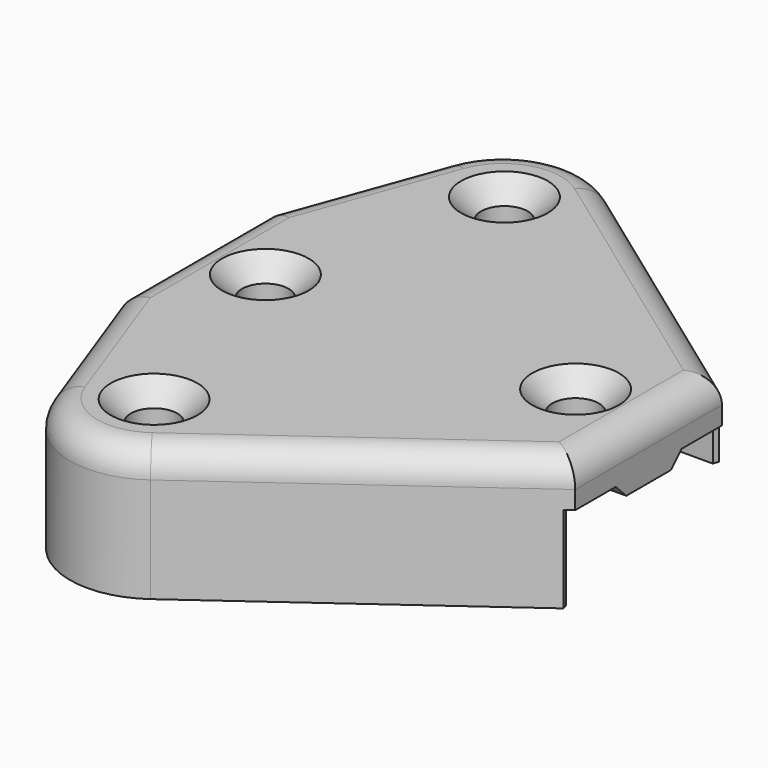
from build123d import *

# Parameters (mm, degrees)
F0_R     = 2.55
F1_DEPTH = 10
F2_W     = 20.1
F2_H     = 5
F3_DEPTH = 50.001
F5_DEPTH = 50
F6_DEPTH = 10
F7_DEPTH = 4.5
F8_DEPTH = 1
F9_R     = 3
F10_SIZE = 2.2
F11_SIZE = 1


# Not quite as in the source:
# - a feature names something its author has since deleted; it is built from what else it names


with BuildPart() as f1:
    # F0 (on Top) → F1 (new body)
    with BuildSketch(Plane.XY):
        with BuildLine():
            Line((-8.8436374201, 26.9644671741), (-15, 10.05))
            Line((-15, 10.05), (-15, -10.05))
            Line((-15, -10.05), (-8.8436374201, -26.9644671741))
            ThreePointArc((-8.8436374201, -26.9644671741), (-2.7616213035, -32.7425446245), (5.5147415904, -31.3718089411))
            Line((5.5147415904, -31.3718089411), (35, -10.05))
            Line((35, -10.05), (35, 10.05))
            Line((35, 10.05), (5.5147415904, 31.3718089411))
            ThreePointArc((5.5147415904, 31.3718089411), (-2.7616213035, 32.7425446245), (-8.8436374201, 26.9644671741))
        make_face()
        with Locations((0, -24)):
            Circle(F0_R, mode=Mode.SUBTRACT)
        with Locations((-7, 0)):
            Circle(F0_R, mode=Mode.SUBTRACT)
        with Locations((0, 24)):
            Circle(F0_R, mode=Mode.SUBTRACT)
        with Locations((27, 0)):
            Circle(F0_R, mode=Mode.SUBTRACT)
    extrude(amount=F1_DEPTH)

    # F2 (on face) → F3 (cut, through all)
    with BuildSketch(Plane(origin=(-15, 0, 0), x_dir=(0, -1, 0), z_dir=(-1, 0, 0))):
        with Locations((0, 2.5)):
            Rectangle(F2_W, F2_H)
    extrude(amount=-F3_DEPTH, mode=Mode.SUBTRACT)

    # F4 (on face) → F5 (join, through all)
    with BuildSketch(Plane(origin=(-15, 0, 0), x_dir=(0, -1, 0), z_dir=(-1, 0, 0))):
        Polygon((3.05, 3.545), (4.5, 5), (-4.5, 5), (-3.05, 3.545), align=None)
    extrude(amount=-F5_DEPTH)

    # F0 (on Top) → F6 (cut, through all)
    with BuildSketch(Plane.XY):
        with Locations((-7, 0)):
            Circle(F0_R)
        with Locations((27, 0)):
            Circle(F0_R)
    extrude(amount=F6_DEPTH, mode=Mode.SUBTRACT)

    # F7 (add): a face of the model
    f7_faces = [f1.faces().sort_by_distance(p)[0] for p in [
        (5.7473624585, -18.668206632, 0),
    ]]
    extrude(f7_faces, amount=F7_DEPTH)

    # F8 (cut): a face of the model
    f8_faces = [f1.faces().sort_by_distance(p)[0] for p in [
        (5.7473624585, 18.668206632, 0),
    ]]
    extrude(f8_faces, amount=-F8_DEPTH, mode=Mode.SUBTRACT)

    # F9
    f9_edges = [f1.edges().sort_by_distance(p)[0] for p in [
        (-11.921819, 18.507234, 10),
        (-15, 0, 10),
        (-11.921819, -18.507234, 10),
        (35, 0, 10),
        (-2.761621, 32.742545, 10),
        (-2.761621, -32.742545, 10),
        (20.257371, -20.710904, 10),
        (20.257371, 20.710904, 10),
    ]]
    fillet(f9_edges, radius=F9_R)

    # F10
    f10_edges = [f1.edges().sort_by_distance(p)[0] for p in [
        (-2.55, -24, 10),
        (-9.55, 0, 10),
        (-2.55, 24, 10),
        (24.45, 0, 10),
    ]]
    chamfer(f10_edges, length=F10_SIZE)

    # F11
    f11_edges = [f1.edges().sort_by_distance(p)[0] for p in [
        (35, 10.05, 3),
        (5.514742, -31.371809, 1.25),
        (35, -10.05, 0.25),
    ]]
    chamfer(f11_edges, length=F11_SIZE)


solid = f1.part
